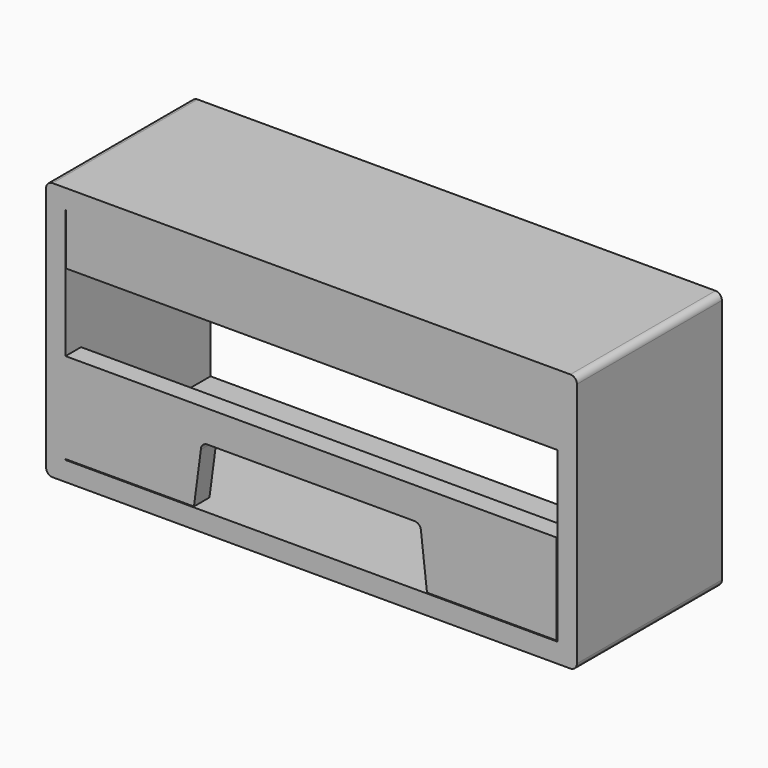
from build123d import *

# Parameters (mm, degrees)
F2_DEPTH = 177.8
F3_DEPTH = 19.05
F1_W     = 482.6
F1_H     = 50.8
F4_DEPTH = 19.05


# Not quite as in the source:
# - a feature names something its author has since deleted; it is built from what else it names


with BuildPart() as f2:
    # F0 (on Front) → F2 (new body)
    with BuildSketch(Plane.XZ):
        with BuildLine():
            Line((-254, -127), (254, -127))
            ThreePointArc((254, -127), (258.4901280605, -125.1401280605), (260.35, -120.65))
            Line((260.35, -120.65), (260.35, 120.65))
            ThreePointArc((260.35, 120.65), (258.4901280605, 125.1401280605), (254, 127))
            Line((254, 127), (-254, 127))
            ThreePointArc((-254, 127), (-258.4901280605, 125.1401280605), (-260.35, 120.65))
            Line((-260.35, 120.65), (-260.35, -120.65))
            ThreePointArc((-260.35, -120.65), (-258.4901280605, -125.1401280605), (-254, -127))
        make_face()
        Polygon((222.25, 107.95), (241.3, 107.95), (241.3, -107.95), (222.25, -107.95), (-222.25, -107.95), (-241.3, -107.95), (-241.3, 107.95), (-222.25, 107.95), align=None, mode=Mode.SUBTRACT)
    extrude(amount=-F2_DEPTH)

    # F1 (on face) → F3 (join)
    with BuildSketch(Plane.XZ):
        Polygon((-222.25, 107.95), (-241.0535812378, 107.95), (-241.0535812378, 57.6071217656), (241.3, 57.6071217656), (241.3, 107.95), (222.25, 107.95), align=None)
    extrude(amount=-F3_DEPTH)

    # F1 (on face) → F4 (join)
    with BuildSketch(Plane.XZ):
        with Locations((0.2464187622, 83.0071217656)):
            Rectangle(F1_W, F1_H)
        with BuildLine():
            Line((-102.1507469177, -49.3358883619), (-0.5507469177, -49.3358883619))
            Line((-0.5507469177, -49.3358883619), (101.0492530823, -49.3358883619))
            ThreePointArc((101.0492530823, -49.3358883619), (105.5393811428, -51.1957603014), (107.3992530823, -55.6858883619))
            Line((107.3992530823, -55.6858883619), (113.2842159033, -107.1381363198))
            Line((113.2842159033, -107.1381363198), (240.2842159033, -107.1381363198))
            Line((240.2842159033, -107.1381363198), (240.2842159033, -18.2381363198))
            Line((240.2842159033, -18.2381363198), (-242.3157840967, -18.2381363198))
            Line((-242.3157840967, -18.2381363198), (-242.3157840967, -107.1381363198))
            Line((-242.3157840967, -107.1381363198), (-115.3157840967, -107.1381363198))
            Line((-115.3157840967, -107.1381363198), (-108.5007469177, -55.6858883619))
            ThreePointArc((-108.5007469177, -55.6858883619), (-106.6408749783, -51.1957603014), (-102.1507469177, -49.3358883619))
        make_face()
    extrude(amount=-F4_DEPTH)


solid = f2.part
